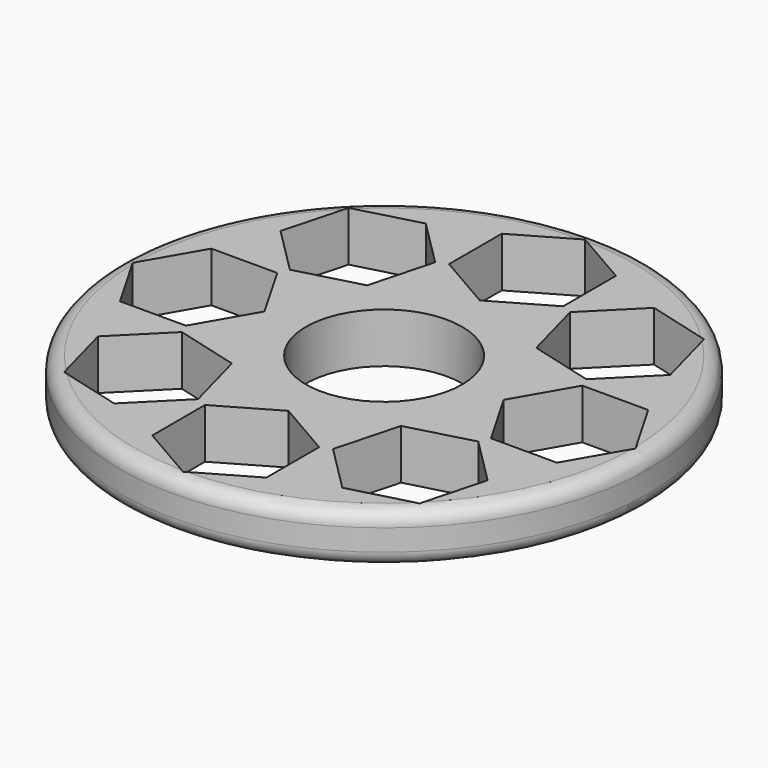
from build123d import *

# Parameters (mm, degrees)
F0_R     = 37
F0_R_2   = 10.95
F1_DEPTH = 7


# Not quite as in the source:
# - a fillet or chamfer that OpenCascade refuses, or shapes differently, is made with other operations: its cross-section is extruded or revolved along the edge and cut away or added


with BuildPart() as f1:
    # F0 (on Top) → F1 (new body)
    with BuildSketch(Plane.XY):
        Circle(F0_R)
        Polygon((-15.9939083851, -27.3076168841), (-24.9167489583, -24.9167489583), (-27.3076168841, -15.9939083851), (-20.7756442366, -9.4619357376), (-11.8528036634, -11.8528036634), (-9.4619357376, -20.7756442366), align=None, mode=Mode.SUBTRACT)
        Polygon((8, -30.6188021535), (0, -35.237604307), (-8, -30.6188021535), (-8, -21.3811978465), (0, -16.762395693), (8, -21.3811978465), align=None, mode=Mode.SUBTRACT)
        Polygon((27.3076168841, -15.9939083851), (24.9167489583, -24.9167489583), (15.9939083851, -27.3076168841), (9.4619357376, -20.7756442366), (11.8528036634, -11.8528036634), (20.7756442366, -9.4619357376), align=None, mode=Mode.SUBTRACT)
        Polygon((-30.6188021535, -8), (-35.237604307, 0), (-30.6188021535, 8), (-21.3811978465, 8), (-16.762395693, 0), (-21.3811978465, -8), align=None, mode=Mode.SUBTRACT)
        Polygon((-27.3076168841, 15.9939083851), (-24.9167489583, 24.9167489583), (-15.9939083851, 27.3076168841), (-9.4619357376, 20.7756442366), (-11.8528036634, 11.8528036634), (-20.7756442366, 9.4619357376), align=None, mode=Mode.SUBTRACT)
        Circle(F0_R_2, mode=Mode.SUBTRACT)
        Polygon((15.9939083851, 27.3076168841), (24.9167489583, 24.9167489583), (27.3076168841, 15.9939083851), (20.7756442366, 9.4619357376), (11.8528036634, 11.8528036634), (9.4619357376, 20.7756442366), align=None, mode=Mode.SUBTRACT)
        Polygon((30.6188021535, 8), (35.237604307, 0), (30.6188021535, -8), (21.3811978465, -8), (16.762395693, 0), (21.3811978465, 8), align=None, mode=Mode.SUBTRACT)
        Polygon((0, 35.237604307), (8, 30.6188021535), (8, 21.3811978465), (0, 16.762395693), (-8, 21.3811978465), (-8, 30.6188021535), align=None, mode=Mode.SUBTRACT)
    extrude(amount=F1_DEPTH)

    # F2: fillet of radius 2 on 2 edges, made by hand

    # F2_s1 → F2_t2 (revolve, cut)
    with BuildSketch(Plane.XZ):
        with BuildLine():
            ThreePointArc((37, 5), (36.4142135624, 6.4142135624), (35, 7))
            Line((35, 7), (37, 7))
            Line((37, 7), (37, 5))
        make_face()
    revolve(axis=Axis((0, 0, 7), (0, 0, 1)), mode=Mode.SUBTRACT)

    # F2_s3 → F2_t4 (revolve, cut)
    with BuildSketch(Plane.XZ):
        with BuildLine():
            ThreePointArc((37, 2), (36.4142135624, 0.5857864376), (35, 0))
            Line((35, 0), (37, 0))
            Line((37, 0), (37, 2))
        make_face()
    revolve(axis=Axis((0, 0, 0), (0, 0, 1)), mode=Mode.SUBTRACT)


solid = f1.part
